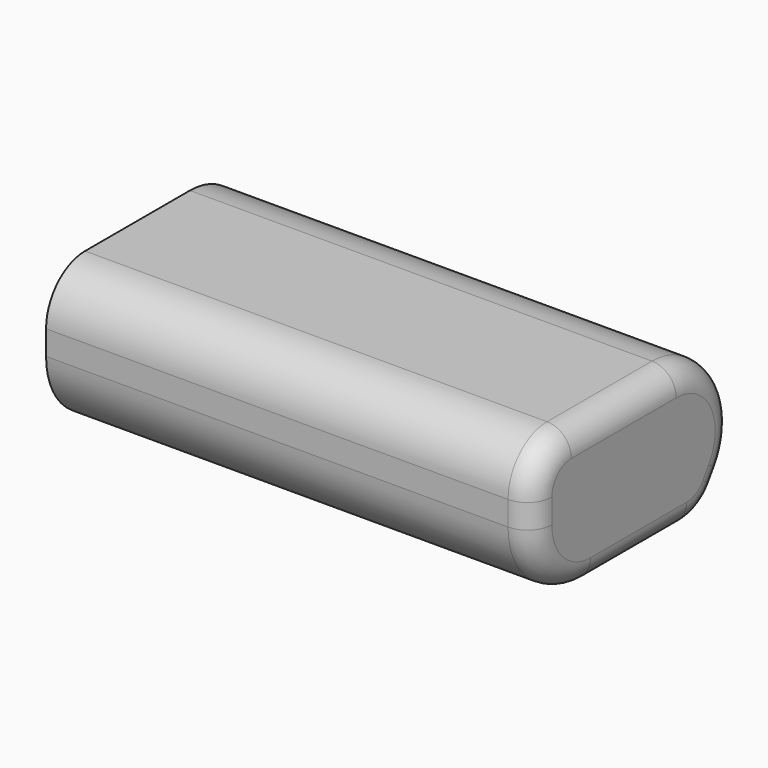
from build123d import *

# Parameters (mm, degrees)
F1_DEPTH = 100
F2_W     = 25
F2_H     = 10
F3_DEPTH = 80
F4_R     = 4.99999
F5_R     = 15
F6_R     = 10
F7_R     = 5


# Not quite as in the source:
# - a fillet or chamfer is up to 0.001 mm smaller than in the source, because OpenCascade refuses the exact size


with BuildPart() as f1:
    # F0 (on Right) → F1 (new body)
    with BuildSketch(Plane.YZ):
        Polygon((65, 0), (0, 0), (0, -30), (45, -30), align=None)
    extrude(amount=F1_DEPTH)

    # F2 (on face) → F3 (cut)
    with BuildSketch(Plane(origin=(0, 0, 0), x_dir=(0, -1, 0), z_dir=(-1, 0, 0))):
        with Locations((-22.5, -15)):
            Rectangle(F2_W, F2_H)
    extrude(amount=-F3_DEPTH, mode=Mode.SUBTRACT)

    # F4 (radius 5 in the source; OpenCascade refuses exactly that, so slightly less here)
    f4_edges = [f1.edges().sort_by_distance(p)[0] for p in [
        (40, 10, -10),
        (40, 35, -10),
        (40, 35, -20),
        (40, 10, -20),
    ]]
    fillet(f4_edges, radius=F4_R)

    # F5
    f5_edges = [f1.edges().sort_by_distance(p)[0] for p in [
        (50, 65, 0),
        (50, 0, -30),
    ]]
    fillet(f5_edges, radius=F5_R)

    # F6
    f6_edges = [f1.edges().sort_by_distance(p)[0] for p in [
        (50, 0, 0),
        (50, 45, -30),
    ]]
    fillet(f6_edges, radius=F6_R)

    # F7
    f7_edges = [f1.edges().sort_by_distance(p)[0] for p in [
        (100, 23.486122, 0),
    ]]
    fillet(f7_edges, radius=F7_R)


solid = f1.part
